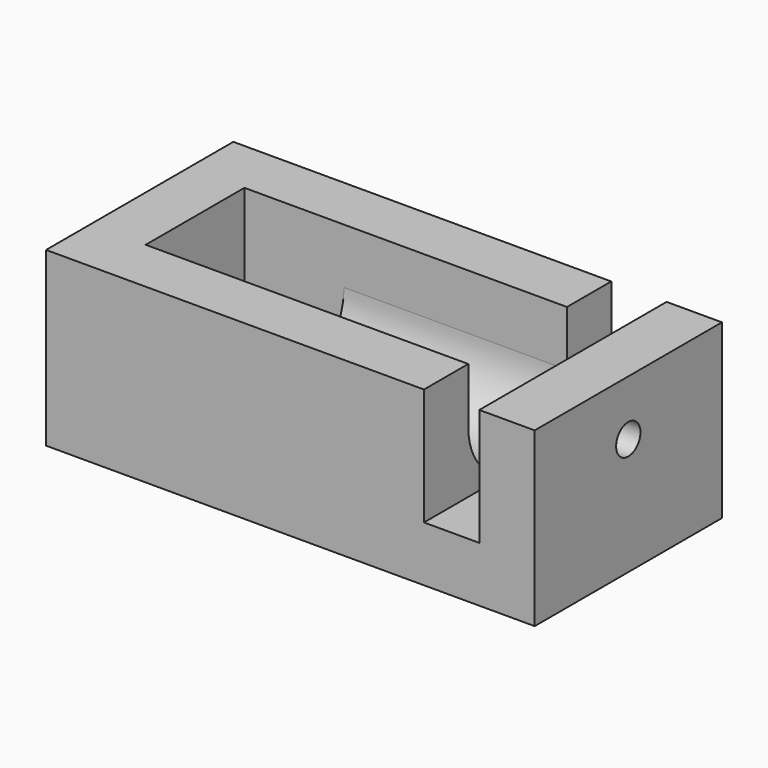
from build123d import *

# Parameters (mm, degrees)
F0_W     = 76.962
F0_H     = 28.321
F0_W_2   = 45.72
F0_W_3   = 25.4
F0_H_2   = 25.4
F1_DEPTH = 53.721
F3_DEPTH = 25.4
F4_DEPTH = 53.721
F5_R     = 6.985
F6_DEPTH = 25.4
F7_DEPTH = 28.321


with BuildPart() as f1:
    # F0 (on Top) → F1 (new body)
    with BuildSketch(Plane.XY):
        Polygon((86.741, -28.321), (61.341, -28.321), (-15.621, -28.321), (-61.341, -28.321), (-61.341, 0), (-61.341, 28.321), (-15.621, 28.321), (61.341, 28.321), (86.741, 28.321), (86.741, 53.721), (-86.741, 53.721), (-86.741, -53.721), (86.741, -53.721), align=None)
        with Locations((22.86, -14.1605)):
            Rectangle(F0_W, F0_H)
        with Locations((-38.481, -14.1605)):
            Rectangle(F0_W_2, F0_H)
        with Locations((74.041, -14.1605)):
            Rectangle(F0_W_3, F0_H)
        with Locations((74.041, 14.1605)):
            Rectangle(F0_W_3, F0_H)
        with Locations((22.86, 14.1605)):
            Rectangle(F0_W, F0_H)
        with Locations((-38.481, 14.1605)):
            Rectangle(F0_W_2, F0_H)
        Polygon((112.141, 0), (112.141, -28.321), (112.141, -53.721), (137.541, -53.721), (137.541, 53.721), (112.141, 53.721), (112.141, 28.321), align=None)
        with Locations((99.441, 41.021)):
            Rectangle(F0_W_3, F0_H_2)
        with Locations((99.441, -41.021)):
            Rectangle(F0_W_3, F0_H_2)
        with Locations((99.441, -14.1605)):
            Rectangle(F0_W_3, F0_H)
        with Locations((99.441, 14.1605)):
            Rectangle(F0_W_3, F0_H)
    extrude(amount=-F1_DEPTH)

    # F0 (on Top) → F2 (revolve, cut)
    with BuildSketch(Plane.XY):
        with Locations((74.041, 14.1605)):
            Rectangle(F0_W_3, F0_H)
        with Locations((-38.481, 14.1605)):
            Rectangle(F0_W_2, F0_H)
        with Locations((22.86, 14.1605)):
            Rectangle(F0_W, F0_H)
    revolve(axis=Axis((0, 0, 0), (1, 0, 0)), mode=Mode.SUBTRACT)

    # F0 (on Top) → F3 (join)
    with BuildSketch(Plane.XY):
        Polygon((86.741, -28.321), (61.341, -28.321), (-15.621, -28.321), (-61.341, -28.321), (-61.341, 0), (-61.341, 28.321), (-15.621, 28.321), (61.341, 28.321), (86.741, 28.321), (86.741, 53.721), (-86.741, 53.721), (-86.741, -53.721), (86.741, -53.721), align=None)
        Polygon((112.141, 0), (112.141, -28.321), (112.141, -53.721), (137.541, -53.721), (137.541, 53.721), (112.141, 53.721), (112.141, 28.321), align=None)
    extrude(amount=F3_DEPTH)

    # F0 (on Top) → F4 (cut)
    with BuildSketch(Plane.XY):
        with Locations((-38.481, 14.1605)):
            Rectangle(F0_W_2, F0_H)
        with Locations((-38.481, -14.1605)):
            Rectangle(F0_W_2, F0_H)
    extrude(amount=-F4_DEPTH, mode=Mode.SUBTRACT)

    # F5 (on face) → F6 (cut)
    with BuildSketch(Plane.YZ.offset(137.541)):
        Circle(F5_R)
    extrude(amount=-F6_DEPTH, mode=Mode.SUBTRACT)

    # F0 (on Top) → F7 (cut)
    with BuildSketch(Plane.XY):
        with Locations((99.441, 41.021)):
            Rectangle(F0_W_3, F0_H_2)
        with Locations((99.441, 14.1605)):
            Rectangle(F0_W_3, F0_H)
        with Locations((99.441, -14.1605)):
            Rectangle(F0_W_3, F0_H)
        with Locations((99.441, -41.021)):
            Rectangle(F0_W_3, F0_H_2)
    extrude(amount=-F7_DEPTH, mode=Mode.SUBTRACT)


solid = f1.part
